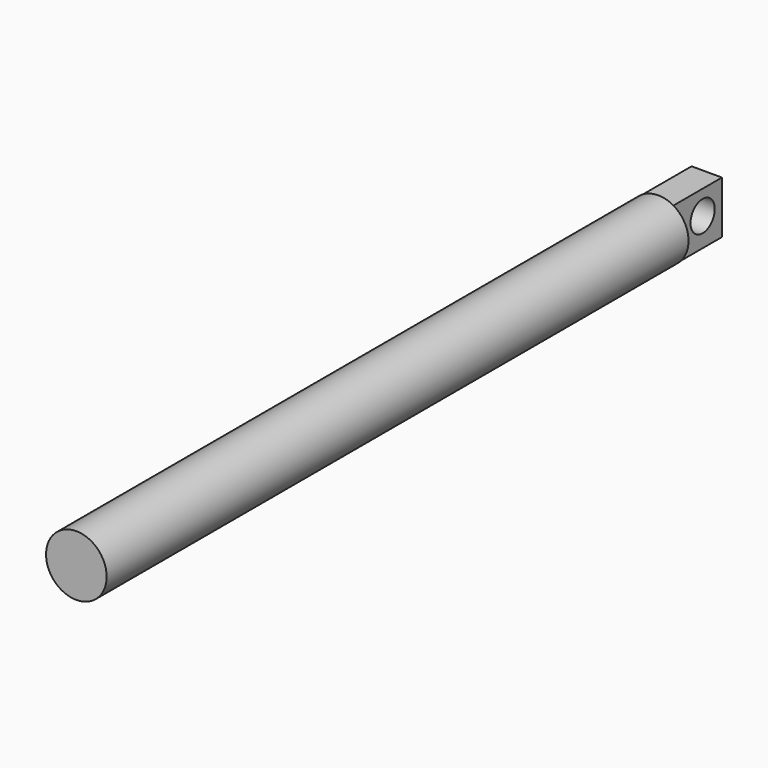
from build123d import *

# Parameters (mm, degrees)
F0_R     = 1.27
F1_DEPTH = 30.48
F3_DEPTH = 2.54
F5_D     = 1.27
F6_R     = 0.5728725826
F7_DEPTH = 0.3302


# Not quite as in the source:
# - a feature names something its author has since deleted; it is built from what else it names


with BuildPart() as f1:
    # F0 (on Front) → F1 (new body)
    with BuildSketch(Plane.XZ):
        with Locations((-44.9135862291, 42.5175279379)):
            Circle(F0_R)
    extrude(amount=F1_DEPTH)

    # F2 (on face) → F3 (join)
    with BuildSketch(Plane(origin=(0, 0, 0), x_dir=(-1, 0, 0), z_dir=(0, 1, 0))):
        Polygon((44.2763268948, 43.6160726756), (44.2763268948, 42.5175279379), (44.2763268948, 41.4189832001), (45.5469042063, 41.4189832001), (45.5469042063, 43.6183496036), align=None)
    extrude(amount=F3_DEPTH)

    # F5 (through all)
    with Locations(Plane(origin=(-45.5469042063, 0, 0), x_dir=(0, -1, 0), z_dir=(-1, 0, 0))):
        with Locations((-1.5291915042, 42.6044538617)):
            Hole(F5_D / 2)

    # F6 (on face) → F7 (cut)
    with BuildSketch(Plane(origin=(0, 2.54, 0), x_dir=(-1, 0, 0), z_dir=(0, 1, 0))):
        with Locations((44.9116155505, 42.5175279379)):
            Circle(F6_R)
    extrude(amount=-F7_DEPTH, mode=Mode.SUBTRACT)


solid = f1.part
